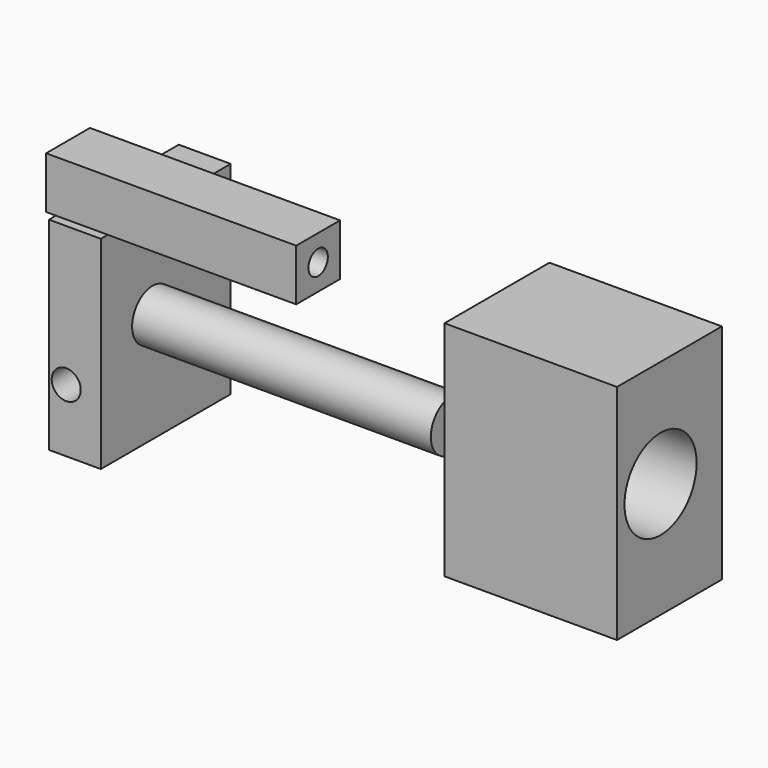
from build123d import *

# Parameters (mm, degrees)
F1_W      = 17.7617222071
F1_H      = 16.7483836412
F1_R      = 3.9272334966
F2_DEPTH  = 81.026
F3_W      = 16.8257057667
F3_H      = 65.6720995903
F3_R      = 4.7053245115
F4_DEPTH  = 25.4
F5_W      = 16.8257057667
F5_H      = 65.6720995903
F5_R      = 4.7053245115
F5_R_2    = 3.4049963351
F6_DEPTH  = 1.778
F9_DEPTH  = 25.4
F12_R     = 8.2733352579
F13_DEPTH = 96.774
F14_W     = 42.485463433
F14_H     = 72.1800103784
F14_R     = 14.6058574256
F15_DEPTH = 55.88


# Not quite as in the source:
# - the program builds the solid bodies; features that only make, move or delete a surface that nothing else refers to are left out


with BuildPart() as f2:
    # F1 (on Right) → F2 (new body)
    with BuildSketch(Plane.YZ):
        with Locations((-65.8714547753, 25.0336769968)):
            Rectangle(F1_W, F1_H)
        with Locations((-65.8714547753, 25.0336769968)):
            Circle(F1_R, mode=Mode.SUBTRACT)
    extrude(amount=F2_DEPTH)


with BuildPart() as f4:
    # F3 (on Front) → F4 (new body)
    with BuildSketch(Plane.XZ):
        with Locations((-8.4128528833, -32.8360497952)):
            Rectangle(F3_W, F3_H)
        with Locations((-11.2144201994, -45.2477447689)):
            Circle(F3_R, mode=Mode.SUBTRACT)
    extrude(amount=F4_DEPTH)

    # F5 (on face) → F6 (join)
    with BuildSketch(Plane.XZ.offset(25.4)):
        with Locations((-8.4128528833, -32.8360497952)):
            Rectangle(F5_W, F5_H)
        with Locations((-11.2144201994, -45.2477447689)):
            Circle(F5_R, mode=Mode.SUBTRACT)
        with Locations((-11.8808113039, -30.071657151)):
            Circle(F5_R_2, mode=Mode.SUBTRACT)
        with Locations((-11.8808113039, -30.071657151)):
            Circle(F5_R_2)
    extrude(amount=F6_DEPTH)

    # F9 (add): a face of the model
    f9_faces = [f4.faces().sort_by_distance(p)[0] for p in [
        (-8.2246562992, -27.178, -32.0022884273),
    ]]
    extrude(f9_faces, amount=F9_DEPTH)

    # F12 (on face) → F13 (join)
    with BuildSketch(Plane.YZ):
        with Locations((-31.6479168832, -30.1750041544)):
            Circle(F12_R)
    extrude(amount=F13_DEPTH)

    # F14 (on face) → F15 (join)
    with BuildSketch(Plane.YZ.offset(96.774)):
        with Locations((-13.1497965194, -36.0900051892)):
            Rectangle(F14_W, F14_H)
        with Locations((-16.7570486665, -34.8301380873)):
            Circle(F14_R, mode=Mode.SUBTRACT)
    extrude(amount=F15_DEPTH)


solid = Compound([f2.part, f4.part])
